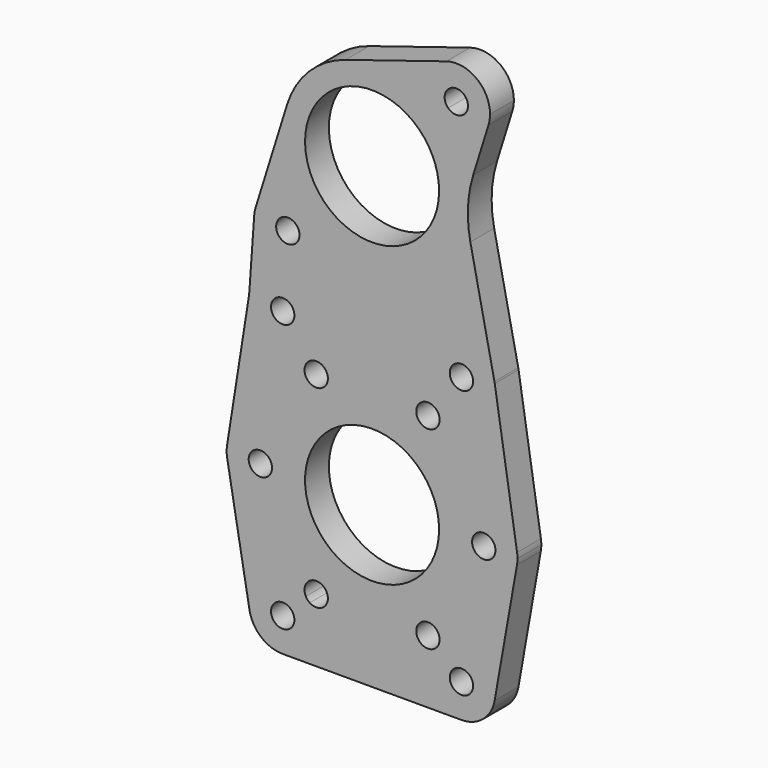
from build123d import *

# Parameters (mm, degrees)
F0_R        = 2.4892
F1_DEPTH    = 6.35
F2_T1_DEPTH = 6.35


# Not quite as in the source:
# - a fillet or chamfer that OpenCascade refuses, or shapes differently, is made with other operations: its cross-section is extruded or revolved along the edge and cut away or added


with BuildPart() as f1:
    # F0 (on Front) → F1 (new body)
    with BuildSketch(Plane.XZ):
        with BuildLine():
            ThreePointArc((13.2773024021, 85.8305287216), (13.0758232734, 85.0225277103), (12.9691446918, 84.1966468751))
            ThreePointArc((12.9691446918, 84.1966468751), (14.0054035794, 79.9428579011), (17.3172773208, 77.0792857545))
            ThreePointArc((17.3172773208, 77.0792857545), (19.6331286406, 76.5199446918), (22.00460406, 76.7482736107))
            ThreePointArc((22.00460406, 76.7482736107), (25.8437426717, 79.3163084348), (27.3276877579, 83.6902877579))
            ThreePointArc((27.3276877579, 83.6902877579), (27.1946025509, 85.0670863985), (26.8002749154, 86.3929038389))
            ThreePointArc((26.8002749154, 86.3929038389), (24.674517099, 88.225317099), (22.8421038389, 90.3510749154))
            ThreePointArc((22.8421038389, 90.3510749154), (17.0679509095, 90.1892015617), (13.2773024021, 85.8305287216))
        make_face()
        with Locations((20.1394877579, 83.6902877579)):
            Circle(F0_R, mode=Mode.SUBTRACT)
        with BuildLine():
            ThreePointArc((26.8002749154, 86.3929038389), (31.0442064849, 84.0240317164), (35.7505, 82.8102312188))
            ThreePointArc((35.7505, 82.8102312188), (38.1, 82.6643), (40.4495, 82.8102312188))
            ThreePointArc((40.4495, 82.8102312188), (42.9672096901, 83.2987578226), (45.3961113108, 84.1221394126))
            ThreePointArc((45.3961113108, 84.1221394126), (47.5091314901, 85.159728875), (49.4775135291, 86.4508207847))
            ThreePointArc((49.4775135291, 86.4508207847), (52.1419442019, 88.8714813453), (54.3015952543, 91.7515326803))
            Line((54.3015952543, 91.7515326803), (54.0915586422, 101.6508))
            Line((54.0915586422, 101.6508), (52.3875, 101.6508))
            ThreePointArc((52.3875, 101.6508), (24.9000711792, 96.1832104601), (48.2027881362, 111.7535881362))
            Line((48.2027881362, 111.7535881362), (50.9776872776, 114.5284872776))
            ThreePointArc((50.9776872776, 114.5284872776), (50.0693141148, 115.6394406129), (49.3997250846, 116.9086961611))
            ThreePointArc((49.3997250846, 116.9086961611), (41.2664943708, 120.3713901523), (32.4468900339, 119.7761835811))
            ThreePointArc((32.4468900339, 119.7761835811), (24.674517099, 115.076282901), (19.9746164189, 107.3039099661))
            ThreePointArc((19.9746164189, 107.3039099661), (19.3794098477, 98.4843056292), (22.8421038389, 90.3510749154))
            ThreePointArc((22.8421038389, 90.3510749154), (25.2223127224, 88.7731127224), (26.8002749154, 86.3929038389))
        make_face()
        with BuildLine():
            ThreePointArc((22.8421038389, 90.3510749154), (24.674517099, 88.225317099), (26.8002749154, 86.3929038389))
            ThreePointArc((26.8002749154, 86.3929038389), (25.2223127224, 88.7731127224), (22.8421038389, 90.3510749154))
        make_face()
        with BuildLine():
            Line((52.3875, 101.6508), (54.0915586422, 101.6508))
            Line((54.0915586422, 101.6508), (53.8671304252, 112.2283602294))
            ThreePointArc((53.8671304252, 112.2283602294), (53.6167151546, 112.5924055979), (53.3578961611, 112.9505250846))
            ThreePointArc((53.3578961611, 112.9505250846), (52.0886406129, 113.6201141148), (50.9776872776, 114.5284872776))
            Line((50.9776872776, 114.5284872776), (48.2027881362, 111.7535881362))
            ThreePointArc((48.2027881362, 111.7535881362), (51.2999288208, 107.1183895399), (52.3875, 101.6508))
        make_face()
        with BuildLine():
            ThreePointArc((51.525482901, 115.076282901), (50.4965080596, 116.03182118), (49.3997250846, 116.9086961611))
            ThreePointArc((49.3997250846, 116.9086961611), (50.0693141148, 115.6394406129), (50.9776872776, 114.5284872776))
            Line((50.9776872776, 114.5284872776), (51.525482901, 115.076282901))
        make_face()
        with BuildLine():
            ThreePointArc((53.3578961611, 112.9505250846), (52.48102118, 114.0473080596), (51.525482901, 115.076282901))
            Line((51.525482901, 115.076282901), (50.9776872776, 114.5284872776))
            ThreePointArc((50.9776872776, 114.5284872776), (52.0886406129, 113.6201141148), (53.3578961611, 112.9505250846))
        make_face()
        with BuildLine():
            ThreePointArc((53.9202712784, 126.4734975979), (49.5615984383, 122.6828490905), (49.3997250846, 116.9086961611))
            ThreePointArc((49.3997250846, 116.9086961611), (50.4965080596, 116.03182118), (51.525482901, 115.076282901))
            ThreePointArc((51.525482901, 115.076282901), (52.48102118, 114.0473080596), (53.3578961611, 112.9505250846))
            ThreePointArc((53.3578961611, 112.9505250846), (53.6051045993, 112.8554856793), (53.8556463568, 112.7696175933))
            ThreePointArc((53.8556463568, 112.7696175933), (56.2129927647, 112.4247296795), (58.5535890214, 112.8692956734))
            ThreePointArc((58.5535890214, 112.8692956734), (61.2734113476, 114.6619787359), (62.9226975979, 117.4710712784))
            ThreePointArc((62.9226975979, 117.4710712784), (63.1667412004, 118.5288478165), (63.2487122421, 119.6113122421))
            ThreePointArc((63.2487122421, 119.6113122421), (60.3199569914, 125.401592863), (53.9202712784, 126.4734975979))
        make_face()
        with BuildLine():
            ThreePointArc((58.5497122421, 119.6113122421), (57.013087842, 117.3115913098), (54.3003820424, 117.8511820424))
            ThreePointArc((54.3003820424, 117.8511820424), (55.1079366423, 121.9110331745), (58.5497122421, 119.6113122421))
        make_face(mode=Mode.SUBTRACT)
        with BuildLine():
            ThreePointArc((22.00460406, 76.7482736107), (19.6331286406, 76.5199446918), (17.3172773208, 77.0792857545))
            Line((17.3172773208, 77.0792857545), (17.1848836978, 75.2045141472))
            ThreePointArc((17.1848836978, 75.2045141472), (19.5563591172, 75.432843066), (21.8722104371, 74.8735020034))
            Line((21.8722104371, 74.8735020034), (22.00460406, 76.7482736107))
        make_face()
        with BuildLine():
            ThreePointArc((11.879656934, 68.7688591172), (12.7603214041, 64.7825341381), (15.6697372294, 61.918680737))
            ThreePointArc((15.6697372294, 61.918680737), (17.4803795527, 61.2477647312), (19.4042866258, 61.0830362159))
            ThreePointArc((19.4042866258, 61.0830362159), (21.8852518822, 64.4761036844), (25.8394633742, 65.9016937117))
            ThreePointArc((25.8394633742, 65.9016937117), (26.1378148913, 67.0653787418), (26.2382, 68.2625))
            ThreePointArc((26.2382, 68.2625), (25.0482010763, 72.2237880592), (21.8722104371, 74.8735020034))
            ThreePointArc((21.8722104371, 74.8735020034), (19.5563591172, 75.432843066), (17.1848836978, 75.2045141472))
            ThreePointArc((17.1848836978, 75.2045141472), (13.7053594795, 73.0692699078), (11.9497622526, 69.3835901706))
            ThreePointArc((11.9497622526, 69.3835901706), (11.9080924989, 69.0769792723), (11.879656934, 68.7688591172))
        make_face()
        with Locations((19.05, 68.2625)):
            Circle(F0_R, mode=Mode.SUBTRACT)
        with BuildLine():
            ThreePointArc((19.4042866258, 61.0830362159), (19.8593939728, 61.1200143937), (20.3112354035, 61.1858126043))
            ThreePointArc((20.3112354035, 61.1858126043), (23.7151175073, 62.7937800508), (25.8394633742, 65.9016937117))
            ThreePointArc((25.8394633742, 65.9016937117), (21.8852518822, 64.4761036844), (19.4042866258, 61.0830362159))
        make_face()
        with BuildLine():
            ThreePointArc((19.5061186901, 56.0867400864), (21.5959350231, 53.1968053577), (24.8175418269, 51.6669999311))
            ThreePointArc((24.8175418269, 51.6669999311), (28.60675, 54.542791329), (32.9918624931, 56.3864461682))
            ThreePointArc((32.9918624931, 56.3864461682), (33.2837574564, 57.5381634141), (33.38195, 58.7222299276))
            ThreePointArc((33.38195, 58.7222299276), (31.1497330567, 63.9288076118), (25.8394633742, 65.9016937117))
            ThreePointArc((25.8394633742, 65.9016937117), (23.7151175073, 62.7937800508), (20.3112354035, 61.1858126043))
            Line((20.3112354035, 61.1858126043), (19.5061186901, 56.0867400864))
        make_face()
        with Locations((26.19375, 58.7222299276)):
            Circle(F0_R, mode=Mode.SUBTRACT)
        with BuildLine():
            ThreePointArc((51.7427044543, 72.9986771632), (50.0943621433, 69.6366155973), (50.3605366258, 65.9016937117))
            ThreePointArc((50.3605366258, 65.9016937117), (54.3147481178, 64.4761036844), (56.7957133742, 61.0830362159))
            ThreePointArc((56.7957133742, 61.0830362159), (58.7196204473, 61.2477647312), (60.5302627706, 61.918680737))
            ThreePointArc((60.5302627706, 61.918680737), (63.3131251848, 64.563026092), (64.3382, 68.2625))
            ThreePointArc((64.3382, 68.2625), (64.3161756961, 68.8247678473), (64.2502377474, 69.3835901706))
            ThreePointArc((64.2502377474, 69.3835901706), (64.2200397807, 69.5604817946), (64.1854355349, 69.7365644741))
            ThreePointArc((64.1854355349, 69.7365644741), (62.4930942353, 73.0709886641), (59.3548658854, 75.1041946488))
            ThreePointArc((59.3548658854, 75.1041946488), (57.6034299499, 75.4363846186), (55.8241066725, 75.3273585353))
            ThreePointArc((55.8241066725, 75.3273585353), (55.2337041191, 75.1905610085), (54.6569232207, 75.0045165687))
            ThreePointArc((54.6569232207, 75.0045165687), (53.0744854744, 74.1836823643), (51.7427044543, 72.9986771632))
        make_face()
        with Locations((57.15, 68.2625)):
            Circle(F0_R, mode=Mode.SUBTRACT)
        with BuildLine():
            ThreePointArc((57.19445, 58.7222299276), (57.0681991156, 57.3809268563), (56.6938813099, 56.0867400864))
            Line((56.6938813099, 56.0867400864), (58.5322372294, 44.443819263))
            ThreePointArc((58.5322372294, 44.443819263), (60.7914098294, 45.2002377474), (63.1737354035, 45.1766873957))
            Line((63.1737354035, 45.1766873957), (60.5302627706, 61.918680737))
            ThreePointArc((60.5302627706, 61.918680737), (58.7196204473, 61.2477647312), (56.7957133742, 61.0830362159))
            ThreePointArc((56.7957133742, 61.0830362159), (57.0940648913, 59.9193511859), (57.19445, 58.7222299276))
        make_face()
        with BuildLine():
            ThreePointArc((57.0865, 38.1), (56.936934824, 35.7215406907), (56.49059568, 33.3805537629))
            ThreePointArc((56.49059568, 33.3805537629), (57.3864626938, 32.5156284558), (58.4181604857, 31.8182955658))
            ThreePointArc((58.4181604857, 31.8182955658), (60.6632962628, 31.0211788225), (63.0456584286, 31.0016782818))
            ThreePointArc((63.0456584286, 31.0016782818), (66.9535512348, 32.9757418402), (68.9913211775, 36.8507962628))
            ThreePointArc((68.9913211775, 36.8507962628), (69.0733030844, 37.4730084323), (69.1007, 38.1))
            ThreePointArc((69.1007, 38.1), (69.0786756961, 38.6622678473), (69.0127377474, 39.2210901706))
            ThreePointArc((69.0127377474, 39.2210901706), (67.0453201693, 43.1323330921), (63.1737354035, 45.1766873957))
            ThreePointArc((63.1737354035, 45.1766873957), (60.7914098294, 45.2002377474), (58.5322372294, 44.443819263))
            ThreePointArc((58.5322372294, 44.443819263), (57.4371024417, 43.7250365275), (56.49059568, 42.8194462371))
            ThreePointArc((56.49059568, 42.8194462371), (56.936934824, 40.4784593093), (57.0865, 38.1))
        make_face()
        with Locations((61.9125, 38.1)):
            Circle(F0_R, mode=Mode.SUBTRACT)
        with BuildLine():
            ThreePointArc((50.3605366258, 65.9016937117), (44.2603204054, 63.0413169069), (43.2081375069, 56.3864461682))
            ThreePointArc((43.2081375069, 56.3864461682), (47.59325, 54.542791329), (51.3824581731, 51.6669999311))
            ThreePointArc((51.3824581731, 51.6669999311), (54.6040649769, 53.1968053577), (56.6938813099, 56.0867400864))
            Line((56.6938813099, 56.0867400864), (55.8887645965, 61.1858126043))
            ThreePointArc((55.8887645965, 61.1858126043), (52.4848824927, 62.7937800508), (50.3605366258, 65.9016937117))
        make_face()
        with Locations((50.00625, 58.7222299276)):
            Circle(F0_R, mode=Mode.SUBTRACT)
        with BuildLine():
            ThreePointArc((19.70940432, 42.8194462371), (21.019659827, 40.6195720477), (21.4757, 38.1))
            ThreePointArc((21.4757, 38.1), (21.019659827, 35.5804279523), (19.70940432, 33.3805537629))
            ThreePointArc((19.70940432, 33.3805537629), (21.657208671, 28.60675), (24.8175418269, 24.5330000689))
            ThreePointArc((24.8175418269, 24.5330000689), (29.78785, 23.7029338799), (32.9918624931, 19.8135538318))
            ThreePointArc((32.9918624931, 19.8135538318), (38.1, 19.1135), (43.2081375069, 19.8135538318))
            ThreePointArc((43.2081375069, 19.8135538318), (46.41215, 23.7029338799), (51.3824581731, 24.5330000689))
            ThreePointArc((51.3824581731, 24.5330000689), (54.542791329, 28.60675), (56.49059568, 33.3805537629))
            ThreePointArc((56.49059568, 33.3805537629), (54.7243, 38.1), (56.49059568, 42.8194462371))
            ThreePointArc((56.49059568, 42.8194462371), (54.542791329, 47.59325), (51.3824581731, 51.6669999311))
            ThreePointArc((51.3824581731, 51.6669999311), (46.41215, 52.4970661201), (43.2081375069, 56.3864461682))
            ThreePointArc((43.2081375069, 56.3864461682), (41.8390977874, 56.7146804965), (40.4495, 56.9405687812))
            ThreePointArc((40.4495, 56.9405687812), (38.1, 57.0865), (35.7505, 56.9405687812))
            ThreePointArc((35.7505, 56.9405687812), (34.3609022126, 56.7146804965), (32.9918624931, 56.3864461682))
            ThreePointArc((32.9918624931, 56.3864461682), (29.78785, 52.4970661201), (24.8175418269, 51.6669999311))
            ThreePointArc((24.8175418269, 51.6669999311), (21.657208671, 47.59325), (19.70940432, 42.8194462371))
        make_face()
        with BuildLine():
            ThreePointArc((23.8125, 38.1), (38.1, 52.3875), (52.3875, 38.1))
            ThreePointArc((52.3875, 38.1), (38.1, 23.8125), (23.8125, 38.1))
        make_face(mode=Mode.SUBTRACT)
        with BuildLine():
            ThreePointArc((56.7957133742, 61.0830362159), (54.3147481178, 64.4761036844), (50.3605366258, 65.9016937117))
            ThreePointArc((50.3605366258, 65.9016937117), (52.4848824927, 62.7937800508), (55.8887645965, 61.1858126043))
            ThreePointArc((55.8887645965, 61.1858126043), (56.3406060272, 61.1200143937), (56.7957133742, 61.0830362159))
        make_face()
        with BuildLine():
            Line((55.8887645965, 61.1858126043), (56.6938813099, 56.0867400864))
            ThreePointArc((56.6938813099, 56.0867400864), (57.0681991156, 57.3809268563), (57.19445, 58.7222299276))
            ThreePointArc((57.19445, 58.7222299276), (57.0940648913, 59.9193511859), (56.7957133742, 61.0830362159))
            ThreePointArc((56.7957133742, 61.0830362159), (56.3406060272, 61.1200143937), (55.8887645965, 61.1858126043))
        make_face()
        with BuildLine():
            ThreePointArc((32.9918624931, 56.3864461682), (28.60675, 54.542791329), (24.8175418269, 51.6669999311))
            ThreePointArc((24.8175418269, 51.6669999311), (29.78785, 52.4970661201), (32.9918624931, 56.3864461682))
        make_face()
        with BuildLine():
            ThreePointArc((13.0262645965, 45.1766873957), (15.4085901706, 45.2002377474), (17.6677627706, 44.443819263))
            Line((17.6677627706, 44.443819263), (19.5061186901, 56.0867400864))
            ThreePointArc((19.5061186901, 56.0867400864), (19.0070425457, 58.5757539709), (19.4042866258, 61.0830362159))
            ThreePointArc((19.4042866258, 61.0830362159), (17.4803795527, 61.2477647312), (15.6697372294, 61.918680737))
            Line((15.6697372294, 61.918680737), (13.0262645965, 45.1766873957))
        make_face()
        with BuildLine():
            ThreePointArc((19.4042866258, 61.0830362159), (19.0070425457, 58.5757539709), (19.5061186901, 56.0867400864))
            Line((19.5061186901, 56.0867400864), (20.3112354035, 61.1858126043))
            ThreePointArc((20.3112354035, 61.1858126043), (19.8593939728, 61.1200143937), (19.4042866258, 61.0830362159))
        make_face()
        with BuildLine():
            ThreePointArc((51.3824581731, 51.6669999311), (47.59325, 54.542791329), (43.2081375069, 56.3864461682))
            ThreePointArc((43.2081375069, 56.3864461682), (46.41215, 52.4970661201), (51.3824581731, 51.6669999311))
        make_face()
        with BuildLine():
            ThreePointArc((56.49059568, 42.8194462371), (54.7243, 38.1), (56.49059568, 33.3805537629))
            ThreePointArc((56.49059568, 33.3805537629), (56.936934824, 35.7215406907), (57.0865, 38.1))
            ThreePointArc((57.0865, 38.1), (56.936934824, 40.4784593093), (56.49059568, 42.8194462371))
        make_face()
        with BuildLine():
            ThreePointArc((19.70940432, 33.3805537629), (19.263065176, 35.7215406907), (19.1135, 38.1))
            ThreePointArc((19.1135, 38.1), (19.263065176, 40.4784593093), (19.70940432, 42.8194462371))
            ThreePointArc((19.70940432, 42.8194462371), (18.7628975583, 43.7250365275), (17.6677627706, 44.443819263))
            ThreePointArc((17.6677627706, 44.443819263), (15.4085901706, 45.2002377474), (13.0262645965, 45.1766873957))
            ThreePointArc((13.0262645965, 45.1766873957), (9.1546798307, 43.1323330921), (7.1872622526, 39.2210901706))
            ThreePointArc((7.1872622526, 39.2210901706), (7.0995933992, 38.0350543392), (7.2086788225, 36.8507962628))
            ThreePointArc((7.2086788225, 36.8507962628), (9.2464487652, 32.9757418402), (13.1543415714, 31.0016782818))
            ThreePointArc((13.1543415714, 31.0016782818), (15.5367037372, 31.0211788225), (17.7818395143, 31.8182955658))
            ThreePointArc((17.7818395143, 31.8182955658), (18.8135373062, 32.5156284558), (19.70940432, 33.3805537629))
        make_face()
        with Locations((14.2875, 38.1)):
            Circle(F0_R, mode=Mode.SUBTRACT)
        with BuildLine():
            Line((19.7502569326, 20.6639301955), (17.7818395143, 31.8182955658))
            ThreePointArc((17.7818395143, 31.8182955658), (15.5367037372, 31.0211788225), (13.1543415714, 31.0016782818))
            Line((13.1543415714, 31.0016782818), (15.5556604857, 17.3942044342))
            ThreePointArc((15.5556604857, 17.3942044342), (17.2463576466, 18.0707392529), (19.0528112327, 18.3006994503))
            ThreePointArc((19.0528112327, 18.3006994503), (19.2995196617, 19.5124217091), (19.7502569326, 20.6639301955))
        make_face()
        with BuildLine():
            ThreePointArc((19.0528112327, 18.3006994503), (17.2463576466, 18.0707392529), (15.5556604857, 17.3942044342))
            ThreePointArc((15.5556604857, 17.3942044342), (12.5595010804, 14.2017787208), (11.9711788225, 9.8632962628))
            ThreePointArc((11.9711788225, 9.8632962628), (14.4298975695, 5.605697591), (19.05, 3.9243))
            ThreePointArc((19.05, 3.9243), (23.2202244148, 5.2576347095), (25.8433842074, 8.763))
            ThreePointArc((25.8433842074, 8.763), (26.0588475271, 9.5167946442), (26.1909387673, 10.2895706221))
            ThreePointArc((26.1909387673, 10.2895706221), (23.542908755, 10.7962088825), (21.2677877423, 12.2427805713))
            ThreePointArc((21.2677877423, 12.2427805713), (21.4703960304, 11.6937053818), (21.5392, 11.1125))
            ThreePointArc((21.5392, 11.1125), (16.8562430855, 9.9362571508), (20.4275599227, 13.1857692298))
            ThreePointArc((20.4275599227, 13.1857692298), (19.2519115156, 15.6120000713), (19.0528112327, 18.3006994503))
        make_face()
        with BuildLine():
            Line((19.1135, 38.1), (21.4757, 38.1))
            ThreePointArc((21.4757, 38.1), (21.019659827, 40.6195720477), (19.70940432, 42.8194462371))
            ThreePointArc((19.70940432, 42.8194462371), (19.263065176, 40.4784593093), (19.1135, 38.1))
        make_face()
        with BuildLine():
            ThreePointArc((32.9918624931, 19.8135538318), (29.78785, 23.7029338799), (24.8175418269, 24.5330000689))
            ThreePointArc((24.8175418269, 24.5330000689), (28.60675, 21.657208671), (32.9918624931, 19.8135538318))
        make_face()
        with BuildLine():
            ThreePointArc((32.9918624931, 19.8135538318), (28.60675, 21.657208671), (24.8175418269, 24.5330000689))
            ThreePointArc((24.8175418269, 24.5330000689), (21.8314848437, 23.1909882501), (19.7502569326, 20.6639301955))
            Line((19.7502569326, 20.6639301955), (20.1831584286, 18.2108217182))
            ThreePointArc((20.1831584286, 18.2108217182), (22.2195800369, 17.5641650277), (23.9759622577, 16.347489501))
            ThreePointArc((23.9759622577, 16.347489501), (25.6125446182, 19.8981661028), (28.68295, 17.4777700724))
            ThreePointArc((28.68295, 17.4777700724), (27.3699928492, 15.2840131579), (24.8161900773, 15.4045008426))
            ThreePointArc((24.8161900773, 15.4045008426), (25.4044515054, 14.4727329243), (25.8433842074, 13.462))
            Line((25.8433842074, 13.462), (32.155612961, 13.462))
            ThreePointArc((32.155612961, 13.462), (33.0685329993, 15.3783468297), (33.38195, 17.4777700724))
            ThreePointArc((33.38195, 17.4777700724), (33.2837574564, 18.6618365859), (32.9918624931, 19.8135538318))
        make_face()
        with BuildLine():
            ThreePointArc((26.1909387673, 10.2895706221), (29.569198328, 11.1313878096), (32.155612961, 13.462))
            Line((32.155612961, 13.462), (25.8433842074, 13.462))
            ThreePointArc((25.8433842074, 13.462), (26.1388089126, 12.3037209871), (26.2382, 11.1125))
            ThreePointArc((26.2382, 11.1125), (26.2263749654, 10.7003573108), (26.1909387673, 10.2895706221))
        make_face()
        with BuildLine():
            Line((20.1831584286, 18.2108217182), (19.7502569326, 20.6639301955))
            ThreePointArc((19.7502569326, 20.6639301955), (19.2995196617, 19.5124217091), (19.0528112327, 18.3006994503))
            ThreePointArc((19.0528112327, 18.3006994503), (19.6197598349, 18.2780839239), (20.1831584286, 18.2108217182))
        make_face()
        with BuildLine():
            ThreePointArc((51.3824581731, 24.5330000689), (46.41215, 23.7029338799), (43.2081375069, 19.8135538318))
            ThreePointArc((43.2081375069, 19.8135538318), (47.59325, 21.657208671), (51.3824581731, 24.5330000689))
        make_face()
        with BuildLine():
            ThreePointArc((51.3838099227, 15.4045008426), (50.7955484946, 14.4727329243), (50.3566157926, 13.462))
            ThreePointArc((50.3566157926, 13.462), (50.004552762, 11.8953173536), (50.0090612327, 10.2895706221))
            ThreePointArc((50.0090612327, 10.2895706221), (52.657091245, 10.7962088825), (54.9322122577, 12.2427805713))
            ThreePointArc((54.9322122577, 12.2427805713), (55.2915226365, 12.7684524538), (55.7724400773, 13.1857692298))
            ThreePointArc((55.7724400773, 13.1857692298), (56.8296929269, 15.2170520751), (57.19445, 17.4777700724))
            ThreePointArc((57.19445, 17.4777700724), (57.1826249654, 17.8899127616), (57.1471887673, 18.3006994503))
            ThreePointArc((57.1471887673, 18.3006994503), (56.5802401651, 18.2780839239), (56.0168415714, 18.2108217182))
            ThreePointArc((56.0168415714, 18.2108217182), (53.9804199631, 17.5641650277), (52.2240377423, 16.347489501))
            ThreePointArc((52.2240377423, 16.347489501), (51.8647273635, 15.8218176185), (51.3838099227, 15.4045008426))
        make_face()
        with BuildLine():
            Line((58.4181604857, 31.8182955658), (56.4497430674, 20.6639301955))
            ThreePointArc((56.4497430674, 20.6639301955), (56.9004803383, 19.5124217091), (57.1471887673, 18.3006994503))
            ThreePointArc((57.1471887673, 18.3006994503), (58.9536423534, 18.0707392529), (60.6443395143, 17.3942044342))
            Line((60.6443395143, 17.3942044342), (63.0456584286, 31.0016782818))
            ThreePointArc((63.0456584286, 31.0016782818), (60.6632962628, 31.0211788225), (58.4181604857, 31.8182955658))
        make_face()
        with BuildLine():
            ThreePointArc((57.1471887673, 18.3006994503), (56.9004803383, 19.5124217091), (56.4497430674, 20.6639301955))
            Line((56.4497430674, 20.6639301955), (56.0168415714, 18.2108217182))
            ThreePointArc((56.0168415714, 18.2108217182), (56.5802401651, 18.2780839239), (57.1471887673, 18.3006994503))
        make_face()
        with BuildLine():
            ThreePointArc((51.3824581731, 24.5330000689), (47.59325, 21.657208671), (43.2081375069, 19.8135538318))
            ThreePointArc((43.2081375069, 19.8135538318), (42.8795535411, 16.5394647794), (44.044387039, 13.462))
            Line((44.044387039, 13.462), (50.3566157926, 13.462))
            ThreePointArc((50.3566157926, 13.462), (50.7955484946, 14.4727329243), (51.3838099227, 15.4045008426))
            ThreePointArc((51.3838099227, 15.4045008426), (47.8124930855, 18.6540129215), (52.49545, 17.4777700724))
            ThreePointArc((52.49545, 17.4777700724), (52.4266460304, 16.8965646905), (52.2240377423, 16.347489501))
            ThreePointArc((52.2240377423, 16.347489501), (53.9804199631, 17.5641650277), (56.0168415714, 18.2108217182))
            Line((56.0168415714, 18.2108217182), (56.4497430674, 20.6639301955))
            ThreePointArc((56.4497430674, 20.6639301955), (54.3685151563, 23.1909882501), (51.3824581731, 24.5330000689))
        make_face()
        with BuildLine():
            Line((50.3566157926, 13.462), (44.044387039, 13.462))
            ThreePointArc((44.044387039, 13.462), (46.630801672, 11.1313878096), (50.0090612327, 10.2895706221))
            ThreePointArc((50.0090612327, 10.2895706221), (50.004552762, 11.8953173536), (50.3566157926, 13.462))
        make_face()
        with BuildLine():
            ThreePointArc((20.1831584286, 18.2108217182), (19.6197598349, 18.2780839239), (19.0528112327, 18.3006994503))
            ThreePointArc((19.0528112327, 18.3006994503), (19.2519115156, 15.6120000713), (20.4275599227, 13.1857692298))
            ThreePointArc((20.4275599227, 13.1857692298), (20.9084773635, 12.7684524538), (21.2677877423, 12.2427805713))
            ThreePointArc((21.2677877423, 12.2427805713), (23.542908755, 10.7962088825), (26.1909387673, 10.2895706221))
            ThreePointArc((26.1909387673, 10.2895706221), (26.2263749654, 10.7003573108), (26.2382, 11.1125))
            ThreePointArc((26.2382, 11.1125), (26.1388089126, 12.3037209871), (25.8433842074, 13.462))
            ThreePointArc((25.8433842074, 13.462), (25.4044515054, 14.4727329243), (24.8161900773, 15.4045008426))
            ThreePointArc((24.8161900773, 15.4045008426), (24.3352726365, 15.8218176185), (23.9759622577, 16.347489501))
            ThreePointArc((23.9759622577, 16.347489501), (22.2195800369, 17.5641650277), (20.1831584286, 18.2108217182))
        make_face()
        with BuildLine():
            ThreePointArc((19.70940432, 33.3805537629), (21.019659827, 35.5804279523), (21.4757, 38.1))
            Line((21.4757, 38.1), (19.1135, 38.1))
            ThreePointArc((19.1135, 38.1), (19.263065176, 35.7215406907), (19.70940432, 33.3805537629))
        make_face()
        with BuildLine():
            ThreePointArc((54.9322122577, 12.2427805713), (52.657091245, 10.7962088825), (50.0090612327, 10.2895706221))
            ThreePointArc((50.0090612327, 10.2895706221), (50.1411524729, 9.5167946442), (50.3566157926, 8.763))
            ThreePointArc((50.3566157926, 8.763), (52.9797755852, 5.2576347095), (57.15, 3.9243))
            ThreePointArc((57.15, 3.9243), (61.7701024305, 5.605697591), (64.2288211775, 9.8632962628))
            ThreePointArc((64.2288211775, 9.8632962628), (64.3108030844, 10.4855084323), (64.3382, 11.1125))
            ThreePointArc((64.3382, 11.1125), (63.3462985135, 14.7561388366), (60.6443395143, 17.3942044342))
            ThreePointArc((60.6443395143, 17.3942044342), (58.9536423534, 18.0707392529), (57.1471887673, 18.3006994503))
            ThreePointArc((57.1471887673, 18.3006994503), (57.1826249654, 17.8899127616), (57.19445, 17.4777700724))
            ThreePointArc((57.19445, 17.4777700724), (56.8296929269, 15.2170520751), (55.7724400773, 13.1857692298))
            ThreePointArc((55.7724400773, 13.1857692298), (58.3262428492, 13.3062569145), (59.6392, 11.1125))
            ThreePointArc((59.6392, 11.1125), (56.5687946182, 8.6921039696), (54.9322122577, 12.2427805713))
        make_face()
        with BuildLine():
            ThreePointArc((50.0090612327, 10.2895706221), (46.630801672, 11.1313878096), (44.044387039, 13.462))
            Line((44.044387039, 13.462), (32.155612961, 13.462))
            ThreePointArc((32.155612961, 13.462), (29.569198328, 11.1313878096), (26.1909387673, 10.2895706221))
            ThreePointArc((26.1909387673, 10.2895706221), (26.0588475271, 9.5167946442), (25.8433842074, 8.763))
            Line((25.8433842074, 8.763), (50.3566157926, 8.763))
            ThreePointArc((50.3566157926, 8.763), (50.1411524729, 9.5167946442), (50.0090612327, 10.2895706221))
        make_face()
        with BuildLine():
            Line((53.8671304252, 112.2283602294), (54.0915586422, 101.6508))
            Line((54.0915586422, 101.6508), (57.0865, 101.6508))
            ThreePointArc((57.0865, 101.6508), (56.9853547603, 103.6079810923), (56.6829966868, 105.5443095208))
            ThreePointArc((56.6829966868, 105.5443095208), (55.5971981077, 109.0220441711), (53.8671304252, 112.2283602294))
        make_face()
        with BuildLine():
            ThreePointArc((53.3578961611, 112.9505250846), (53.6167151546, 112.5924055979), (53.8671304252, 112.2283602294))
            Line((53.8671304252, 112.2283602294), (53.8556463568, 112.7696175933))
            ThreePointArc((53.8556463568, 112.7696175933), (53.6051045993, 112.8554856793), (53.3578961611, 112.9505250846))
        make_face()
        with BuildLine():
            Line((35.7505, 82.8102312188), (35.7505, 56.9405687812))
            ThreePointArc((35.7505, 56.9405687812), (38.1, 57.0865), (40.4495, 56.9405687812))
            Line((40.4495, 56.9405687812), (40.4495, 82.8102312188))
            ThreePointArc((40.4495, 82.8102312188), (38.1, 82.6643), (35.7505, 82.8102312188))
        make_face()
        with BuildLine():
            ThreePointArc((49.4775135291, 86.4508207847), (47.5091314901, 85.159728875), (45.3961113108, 84.1221394126))
            Line((45.3961113108, 84.1221394126), (51.7427044543, 72.9986771632))
            ThreePointArc((51.7427044543, 72.9986771632), (53.0744854744, 74.1836823643), (54.6569232207, 75.0045165687))
            Line((54.6569232207, 75.0045165687), (54.60472832, 77.4645223279))
            Line((54.60472832, 77.4645223279), (49.4775135291, 86.4508207847))
        make_face()
        with BuildLine():
            Line((54.60472832, 77.4645223279), (54.6569232207, 75.0045165687))
            ThreePointArc((54.6569232207, 75.0045165687), (55.2337041191, 75.1905610085), (55.8241066725, 75.3273585353))
            Line((55.8241066725, 75.3273585353), (54.60472832, 77.4645223279))
        make_face()
        with BuildLine():
            Line((54.0915586422, 101.6508), (54.3015952543, 91.7515326803))
            ThreePointArc((54.3015952543, 91.7515326803), (55.3943005658, 93.8153453105), (56.2253835811, 95.9976900339))
            ThreePointArc((56.2253835811, 95.9976900339), (56.8699863827, 98.7916404305), (57.0865, 101.6508))
            Line((57.0865, 101.6508), (54.0915586422, 101.6508))
        make_face()
        with BuildLine():
            Line((53.9202712784, 126.4734975979), (32.4468900339, 119.7761835811))
            ThreePointArc((32.4468900339, 119.7761835811), (41.2664943708, 120.3713901523), (49.3997250846, 116.9086961611))
            ThreePointArc((49.3997250846, 116.9086961611), (49.5615984383, 122.6828490905), (53.9202712784, 126.4734975979))
        make_face()
        with BuildLine():
            Line((19.9746164189, 107.3039099661), (13.2773024021, 85.8305287216))
            ThreePointArc((13.2773024021, 85.8305287216), (17.0679509095, 90.1892015617), (22.8421038389, 90.3510749154))
            ThreePointArc((22.8421038389, 90.3510749154), (19.3794098477, 98.4843056292), (19.9746164189, 107.3039099661))
        make_face()
        with BuildLine():
            Line((12.9691446918, 84.1966468751), (11.9014692679, 69.0777346006))
            Line((11.9014692679, 69.0777346006), (11.9497622526, 69.3835901706))
            ThreePointArc((11.9497622526, 69.3835901706), (13.7053594795, 73.0692699078), (17.1848836978, 75.2045141472))
            Line((17.1848836978, 75.2045141472), (17.3172773208, 77.0792857545))
            ThreePointArc((17.3172773208, 77.0792857545), (14.0054035794, 79.9428579011), (12.9691446918, 84.1966468751))
        make_face()
        with BuildLine():
            ThreePointArc((7.1872622526, 39.2210901706), (9.1546798307, 43.1323330921), (13.0262645965, 45.1766873957))
            Line((13.0262645965, 45.1766873957), (15.6697372294, 61.918680737))
            ThreePointArc((15.6697372294, 61.918680737), (12.7603214041, 64.7825341381), (11.879656934, 68.7688591172))
            Line((11.879656934, 68.7688591172), (11.9014692679, 69.0777346006))
            Line((11.9014692679, 69.0777346006), (7.1872622526, 39.2210901706))
        make_face()
        with BuildLine():
            ThreePointArc((25.8433842074, 8.763), (23.2202244148, 5.2576347095), (19.05, 3.9243))
            Line((19.05, 3.9243), (57.15, 3.9243))
            ThreePointArc((57.15, 3.9243), (52.9797755852, 5.2576347095), (50.3566157926, 8.763))
            Line((50.3566157926, 8.763), (25.8433842074, 8.763))
        make_face()
        with BuildLine():
            ThreePointArc((64.3382, 11.1125), (64.3108030844, 10.4855084323), (64.2288211775, 9.8632962628))
            Line((64.2288211775, 9.8632962628), (68.9913211775, 36.8507962628))
            ThreePointArc((68.9913211775, 36.8507962628), (66.9535512348, 32.9757418402), (63.0456584286, 31.0016782818))
            Line((63.0456584286, 31.0016782818), (60.6443395143, 17.3942044342))
            ThreePointArc((60.6443395143, 17.3942044342), (63.3462985135, 14.7561388366), (64.3382, 11.1125))
        make_face()
        with BuildLine():
            ThreePointArc((64.3382, 68.2625), (63.3131251848, 64.563026092), (60.5302627706, 61.918680737))
            Line((60.5302627706, 61.918680737), (63.1737354035, 45.1766873957))
            ThreePointArc((63.1737354035, 45.1766873957), (67.0453201693, 43.1323330921), (69.0127377474, 39.2210901706))
            Line((69.0127377474, 39.2210901706), (64.2502377474, 69.3835901706))
            ThreePointArc((64.2502377474, 69.3835901706), (64.3161756961, 68.8247678473), (64.3382, 68.2625))
        make_face()
        with BuildLine():
            Line((58.9372909435, 94.7849823688), (59.3548658854, 75.1041946488))
            ThreePointArc((59.3548658854, 75.1041946488), (62.4930942353, 73.0709886641), (64.1854355349, 69.7365644741))
            Line((64.1854355349, 69.7365644741), (58.9372909435, 94.7849823688))
        make_face()
        with BuildLine():
            Line((58.7404630424, 104.0617079368), (62.9226975979, 117.4710712784))
            ThreePointArc((62.9226975979, 117.4710712784), (61.2734113476, 114.6619787359), (58.5535890214, 112.8692956734))
            Line((58.5535890214, 112.8692956734), (58.7404630424, 104.0617079368))
        make_face()
        with BuildLine():
            Line((53.8556463568, 112.7696175933), (53.8671304252, 112.2283602294))
            ThreePointArc((53.8671304252, 112.2283602294), (55.5971981077, 109.0220441711), (56.6829966868, 105.5443095208))
            Line((56.6829966868, 105.5443095208), (57.4987648131, 101.6508))
            Line((57.4987648131, 101.6508), (57.9885270834, 101.6508))
            Line((57.9885270834, 101.6508), (58.7404630424, 104.0617079368))
            Line((58.7404630424, 104.0617079368), (58.5535890214, 112.8692956734))
            ThreePointArc((58.5535890214, 112.8692956734), (56.2129927647, 112.4247296795), (53.8556463568, 112.7696175933))
        make_face()
        with BuildLine():
            ThreePointArc((56.2253835811, 95.9976900339), (55.3943005658, 93.8153453105), (54.3015952543, 91.7515326803))
            Line((54.3015952543, 91.7515326803), (54.60472832, 77.4645223279))
            Line((54.60472832, 77.4645223279), (55.8241066725, 75.3273585353))
            ThreePointArc((55.8241066725, 75.3273585353), (57.6034299499, 75.4363846186), (59.3548658854, 75.1041946488))
            Line((59.3548658854, 75.1041946488), (58.9372909435, 94.7849823688))
            Line((58.9372909435, 94.7849823688), (57.6955680286, 100.711494861))
            Line((57.6955680286, 100.711494861), (56.2253835811, 95.9976900339))
        make_face()
        with BuildLine():
            ThreePointArc((54.3015952543, 91.7515326803), (52.1419442019, 88.8714813453), (49.4775135291, 86.4508207847))
            Line((49.4775135291, 86.4508207847), (54.60472832, 77.4645223279))
            Line((54.60472832, 77.4645223279), (54.3015952543, 91.7515326803))
        make_face()
        with BuildLine():
            Line((40.4495, 82.8102312188), (40.4495, 56.9405687812))
            ThreePointArc((40.4495, 56.9405687812), (41.8390977874, 56.7146804965), (43.2081375069, 56.3864461682))
            ThreePointArc((43.2081375069, 56.3864461682), (44.2603204054, 63.0413169069), (50.3605366258, 65.9016937117))
            ThreePointArc((50.3605366258, 65.9016937117), (50.0943621433, 69.6366155973), (51.7427044543, 72.9986771632))
            Line((51.7427044543, 72.9986771632), (45.3961113108, 84.1221394126))
            ThreePointArc((45.3961113108, 84.1221394126), (42.9672096901, 83.2987578226), (40.4495, 82.8102312188))
        make_face()
        with BuildLine():
            ThreePointArc((33.38195, 58.7222299276), (33.2837574564, 57.5381634141), (32.9918624931, 56.3864461682))
            ThreePointArc((32.9918624931, 56.3864461682), (34.3609022126, 56.7146804965), (35.7505, 56.9405687812))
            Line((35.7505, 56.9405687812), (35.7505, 82.8102312188))
            ThreePointArc((35.7505, 82.8102312188), (31.0442064849, 84.0240317164), (26.8002749154, 86.3929038389))
            ThreePointArc((26.8002749154, 86.3929038389), (27.1946025509, 85.0670863985), (27.3276877579, 83.6902877579))
            ThreePointArc((27.3276877579, 83.6902877579), (25.8437426717, 79.3163084348), (22.00460406, 76.7482736107))
            Line((22.00460406, 76.7482736107), (21.8722104371, 74.8735020034))
            ThreePointArc((21.8722104371, 74.8735020034), (25.0482010763, 72.2237880592), (26.2382, 68.2625))
            ThreePointArc((26.2382, 68.2625), (26.1378148913, 67.0653787418), (25.8394633742, 65.9016937117))
            ThreePointArc((25.8394633742, 65.9016937117), (31.1497330567, 63.9288076118), (33.38195, 58.7222299276))
        make_face()
        with BuildLine():
            ThreePointArc((17.6677627706, 44.443819263), (18.7628975583, 43.7250365275), (19.70940432, 42.8194462371))
            ThreePointArc((19.70940432, 42.8194462371), (21.657208671, 47.59325), (24.8175418269, 51.6669999311))
            ThreePointArc((24.8175418269, 51.6669999311), (21.5959350231, 53.1968053577), (19.5061186901, 56.0867400864))
            Line((19.5061186901, 56.0867400864), (17.6677627706, 44.443819263))
        make_face()
        with BuildLine():
            ThreePointArc((56.6938813099, 56.0867400864), (54.6040649769, 53.1968053577), (51.3824581731, 51.6669999311))
            ThreePointArc((51.3824581731, 51.6669999311), (54.542791329, 47.59325), (56.49059568, 42.8194462371))
            ThreePointArc((56.49059568, 42.8194462371), (57.4371024417, 43.7250365275), (58.5322372294, 44.443819263))
            Line((58.5322372294, 44.443819263), (56.6938813099, 56.0867400864))
        make_face()
        with BuildLine():
            ThreePointArc((56.49059568, 33.3805537629), (54.542791329, 28.60675), (51.3824581731, 24.5330000689))
            ThreePointArc((51.3824581731, 24.5330000689), (54.3685151563, 23.1909882501), (56.4497430674, 20.6639301955))
            Line((56.4497430674, 20.6639301955), (58.4181604857, 31.8182955658))
            ThreePointArc((58.4181604857, 31.8182955658), (57.3864626938, 32.5156284558), (56.49059568, 33.3805537629))
        make_face()
        with BuildLine():
            ThreePointArc((43.2081375069, 19.8135538318), (38.1, 19.1135), (32.9918624931, 19.8135538318))
            ThreePointArc((32.9918624931, 19.8135538318), (33.2837574564, 18.6618365859), (33.38195, 17.4777700724))
            ThreePointArc((33.38195, 17.4777700724), (33.0685329993, 15.3783468297), (32.155612961, 13.462))
            Line((32.155612961, 13.462), (44.044387039, 13.462))
            ThreePointArc((44.044387039, 13.462), (42.8795535411, 16.5394647794), (43.2081375069, 19.8135538318))
        make_face()
        with BuildLine():
            ThreePointArc((24.8175418269, 24.5330000689), (21.657208671, 28.60675), (19.70940432, 33.3805537629))
            ThreePointArc((19.70940432, 33.3805537629), (18.8135373062, 32.5156284558), (17.7818395143, 31.8182955658))
            Line((17.7818395143, 31.8182955658), (19.7502569326, 20.6639301955))
            ThreePointArc((19.7502569326, 20.6639301955), (21.8314848437, 23.1909882501), (24.8175418269, 24.5330000689))
        make_face()
        Polygon((57.4987648131, 101.6508), (57.6955680286, 100.711494861), (57.9885270834, 101.6508), align=None)
        with BuildLine():
            ThreePointArc((57.0865, 101.6508), (56.8699863827, 98.7916404305), (56.2253835811, 95.9976900339))
            Line((56.2253835811, 95.9976900339), (57.6955680286, 100.711494861))
            Line((57.6955680286, 100.711494861), (57.4987648131, 101.6508))
            Line((57.4987648131, 101.6508), (57.0865, 101.6508))
        make_face()
        with BuildLine():
            ThreePointArc((56.6829966868, 105.5443095208), (56.9853547603, 103.6079810923), (57.0865, 101.6508))
            Line((57.0865, 101.6508), (57.4987648131, 101.6508))
            Line((57.4987648131, 101.6508), (56.6829966868, 105.5443095208))
        make_face()
        with BuildLine():
            Line((15.5556604857, 17.3942044342), (13.1543415714, 31.0016782818))
            ThreePointArc((13.1543415714, 31.0016782818), (9.2464487652, 32.9757418402), (7.2086788225, 36.8507962628))
            Line((7.2086788225, 36.8507962628), (11.9711788225, 9.8632962628))
            ThreePointArc((11.9711788225, 9.8632962628), (12.5595010804, 14.2017787208), (15.5556604857, 17.3942044342))
        make_face()
        with BuildLine():
            Line((11.9497622526, 69.3835901706), (11.9014692679, 69.0777346006))
            Line((11.9014692679, 69.0777346006), (11.879656934, 68.7688591172))
            ThreePointArc((11.879656934, 68.7688591172), (11.9080924989, 69.0769792723), (11.9497622526, 69.3835901706))
        make_face()
    extrude(amount=F1_DEPTH)

    # F2: fillet of radius 25.4 on 17 edges, made by hand

    # F2_s2 → F2_t1 (join)
    with BuildSketch(Plane.XZ):
        with BuildLine():
            ThreePointArc((11.9785446527, 70.1691674039), (11.8780656248, 69.0804036049), (11.7308226787, 67.9969728689))
            Line((11.7308226787, 67.9969728689), (11.9014692679, 69.0777346006))
            Line((11.9014692679, 69.0777346006), (11.9785446527, 70.1691674039))
        make_face()
        with BuildLine():
            ThreePointArc((59.0501785193, 94.2461909684), (58.5395056472, 100.6710410737), (59.6623699651, 107.0175882752))
            Line((59.6623699651, 107.0175882752), (57.6955680286, 100.711494861))
            Line((57.6955680286, 100.711494861), (59.0501785193, 94.2461909684))
        make_face()
    extrude(amount=F2_T1_DEPTH)


solid = f1.part
